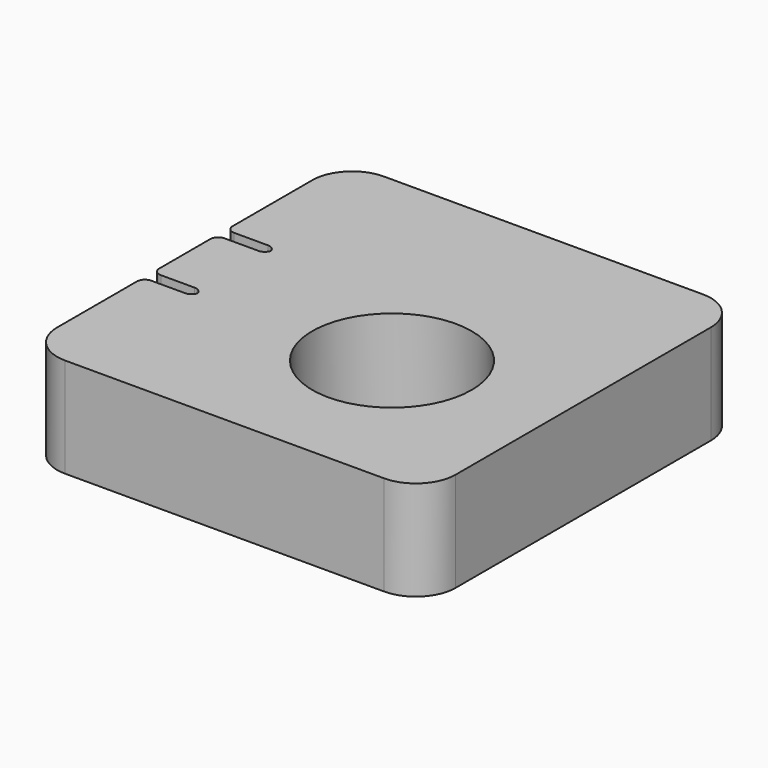
from build123d import *

# Parameters (mm, degrees)
F0_W        = 20
F0_H        = 20
F1_DEPTH    = 5
F2_W        = 3.5
F2_H        = 16.5
F3_DEPTH    = 1.2
F4_R        = 4
F5_DEPTH    = 5.001
F6_R        = 2
F7_W        = 0.6
F7_H        = 3.8
F8_DEPTH    = 2.5
F9_T1_DEPTH = 3.8
F9_T3_DEPTH = 5.8


# Not quite as in the source:
# - a fillet or chamfer that OpenCascade refuses, or shapes differently, is made with other operations: its cross-section is extruded or revolved along the edge and cut away or added


with BuildPart() as f1:
    # F0 (on Top) → F1 (new body)
    with BuildSketch(Plane.XY):
        Rectangle(F0_W, F0_H)
    extrude(amount=F1_DEPTH)

    # F2 (on face) → F3 (cut)
    with BuildSketch(Plane(origin=(0, 0, 0), x_dir=(1, 0, 0), z_dir=(0, 0, -1))):
        with Locations((-8.25, -1.75)):
            Rectangle(F2_W, F2_H)
    extrude(amount=-F3_DEPTH, mode=Mode.SUBTRACT)

    # F4 (on face) → F5 (cut, through all)
    with BuildSketch(Plane.XY.offset(5)):
        with Locations((2, -2)):
            Circle(F4_R)
    extrude(amount=-F5_DEPTH, mode=Mode.SUBTRACT)

    # F6
    f6_edges = [f1.edges().sort_by_distance(p)[0] for p in [
        (10, -10, 2.5),
        (-10, -10, 2.5),
        (-10, 10, 3.1),
        (10, 10, 2.5),
    ]]
    fillet(f6_edges, radius=F6_R)

    # F7 (on face) → F8 (cut)
    with BuildSketch(Plane(origin=(-10, 0, 0), x_dir=(0, -1, 0), z_dir=(-1, 0, 0))):
        with Locations((-2.3, 3.1)):
            Rectangle(F7_W, F7_H)
        with Locations((2.3, 3.1)):
            Rectangle(F7_W, F7_H)
    extrude(amount=-F8_DEPTH, mode=Mode.SUBTRACT)

    # F9: fillet of radius 0.4 on 8 edges, made by hand

    # F9_s2 → F9_t1 (join)
    with BuildSketch(Plane.XY.offset(1.2)):
        with BuildLine():
            ThreePointArc((-7.5, 2.2), (-7.6171572875, 2.4828427125), (-7.9, 2.6))
            Line((-7.9, 2.6), (-7.5, 2.6))
            Line((-7.5, 2.6), (-7.5, 2.2))
        make_face()
        with BuildLine():
            ThreePointArc((-7.9, 2), (-7.6171572875, 2.1171572875), (-7.5, 2.4))
            Line((-7.5, 2.4), (-7.5, 2))
            Line((-7.5, 2), (-7.9, 2))
        make_face()
        with BuildLine():
            ThreePointArc((-7.9, -2.6), (-7.6171572875, -2.4828427125), (-7.5, -2.2))
            Line((-7.5, -2.2), (-7.5, -2.6))
            Line((-7.5, -2.6), (-7.9, -2.6))
        make_face()
        with BuildLine():
            ThreePointArc((-7.5, -2.4), (-7.6171572875, -2.1171572875), (-7.9, -2))
            Line((-7.9, -2), (-7.5, -2))
            Line((-7.5, -2), (-7.5, -2.4))
        make_face()
    extrude(amount=F9_T1_DEPTH)

    # F9_s4 → F9_t3 (cut)
    with BuildSketch(Plane.XY.offset(0.2)):
        with BuildLine():
            ThreePointArc((-10, 1.6), (-9.8828427125, 1.8828427125), (-9.6, 2))
            Line((-9.6, 2), (-10, 2))
            Line((-10, 2), (-10, 1.6))
        make_face()
        with BuildLine():
            ThreePointArc((-9.6, -2), (-9.8828427125, -1.8828427125), (-10, -1.6))
            Line((-10, -1.6), (-10, -2))
            Line((-10, -2), (-9.6, -2))
        make_face()
        with BuildLine():
            ThreePointArc((-10, -3), (-9.8828427125, -2.7171572875), (-9.6, -2.6))
            Line((-9.6, -2.6), (-10, -2.6))
            Line((-10, -2.6), (-10, -3))
        make_face()
        with BuildLine():
            ThreePointArc((-9.6, 2.6), (-9.8828427125, 2.7171572875), (-10, 3))
            Line((-10, 3), (-10, 2.6))
            Line((-10, 2.6), (-9.6, 2.6))
        make_face()
    extrude(amount=F9_T3_DEPTH, mode=Mode.SUBTRACT)


solid = f1.part
